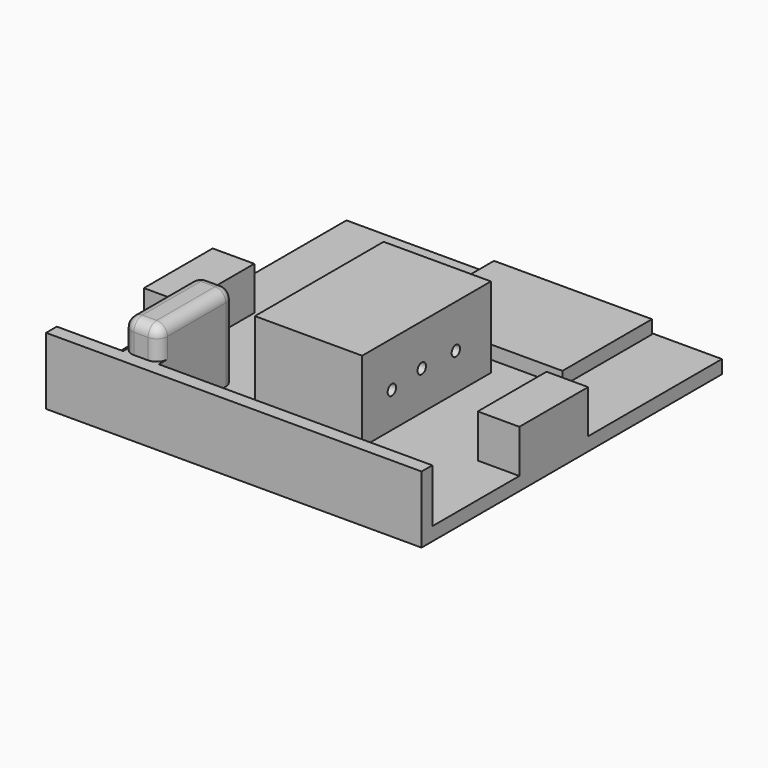
from build123d import *

# Parameters (mm, degrees)
F0_W      = 177.8
F0_H      = 177.8
F1_DEPTH  = 6.35
F2_W      = 19.7
F2_H      = 40.7
F3_DEPTH  = 20.5
F4_W      = 50.8
F4_H      = 76.2
F5_DEPTH  = 38.1
F6_W      = 74.8
F6_H      = 53
F7_DEPTH  = 6.35
F8_W      = 177.8
F8_H      = 6.35
F9_DEPTH  = 25.4
F10_W     = 16.9
F10_H     = 44.7
F11_DEPTH = 40
F13_D     = 5
F13_DEPTH = 12.7
F13_TIP   = 1.5021515476
F14_R     = 5.08


# Not quite as in the source:
# - a feature of the source that left no trace in its solid (it failed there, or was rolled back) is left out


with BuildPart() as f1:
    # F0 (on Top) → F1 (new body)
    with BuildSketch(Plane.XY):
        with Locations((-29.0734948754, -26.9331749929)):
            Rectangle(F0_W, F0_H)
    extrude(amount=F1_DEPTH)

    # F2 (on face) → F3 (join)
    with BuildSketch(Plane.XY.offset(6.35)):
        with Locations((49.9765051246, -37.5782008111)):
            Rectangle(F2_W, F2_H)
        with Locations((-108.1234948754, -37.5782008111)):
            Rectangle(F2_W, F2_H)
    extrude(amount=F3_DEPTH)

    # F4 (on face) → F5 (join)
    with BuildSketch(Plane.XY.offset(6.35)):
        with Locations((-25.4, -38.1)):
            Rectangle(F4_W, F4_H)
    extrude(amount=F5_DEPTH)

    # F6 (on face) → F7 (join)
    with BuildSketch(Plane.XY.offset(6.35)):
        with Locations((-10.0883172065, 34.7147134863)):
            Rectangle(F6_W, F6_H)
    extrude(amount=F7_DEPTH)

    # F8 (on face) → F9 (join)
    with BuildSketch(Plane.XY.offset(6.35)):
        with Locations((-29.0734948754, -112.6581749929)):
            Rectangle(F8_W, F8_H)
    extrude(amount=F9_DEPTH)

    # F10 (on face) → F11 (join)
    with BuildSketch(Plane.XY.offset(6.35)):
        with Locations((-78.1089827299, -87.1331749929)):
            Rectangle(F10_W, F10_H)
    extrude(amount=F11_DEPTH)

    # F13 (one way)
    with BuildSketch(Plane.YZ):
        with Locations((-58.6075335741, 23.0651237071), (-40.9188605845, 24.820599705), (-20.7475721836, 23.942861706)):
            Circle(F13_D / 2)
    extrude(amount=-F13_DEPTH, mode=Mode.SUBTRACT)
    with Locations(Plane.YZ):
        with Locations((-58.6075335741, 23.0651237071), (-40.9188605845, 24.820599705), (-20.7475721836, 23.942861706)):
            with Locations((0, 0, -(F13_DEPTH + F13_TIP / 2))):  # 118° drill point
                Cone(0, F13_D / 2, F13_TIP, mode=Mode.SUBTRACT)

    # F14
    f14_edges = [f1.edges().sort_by_distance(p)[0] for p in [
        (-69.658983, -87.133175, 46.35),
        (-78.108983, -64.783175, 46.35),
        (-86.558983, -87.133175, 46.35),
        (-78.108983, -109.483175, 46.35),
        (-86.558983, -64.783175, 26.35),
        (-69.658983, -64.783175, 26.35),
        (-69.658983, -109.483175, 39.05),
        (-86.558983, -109.483175, 39.05),
    ]]
    fillet(f14_edges, radius=F14_R)


solid = f1.part
